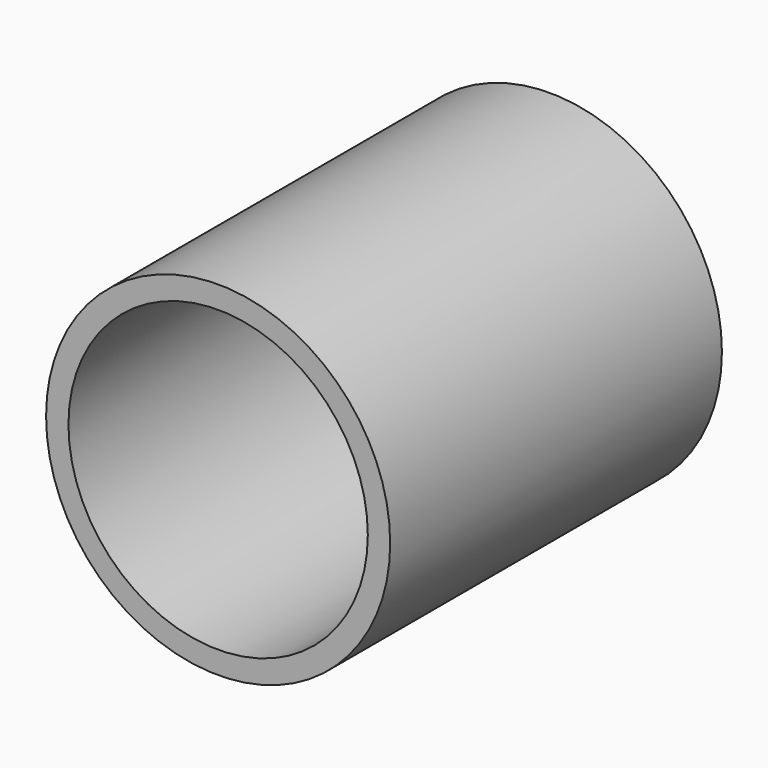
from build123d import *

# Parameters (mm, degrees)
F0_R     = 42.1551609163
F0_R_2   = 36.6737913898
F1_DEPTH = 101.6
F2_R     = 36.6906853339
F3_DEPTH = 0.254


# Not quite as in the source:
# - the program builds the solid bodies; features that only make, move or delete a surface that nothing else refers to are left out


with BuildPart() as f1:
    # F0 (on Front) → F1 (new body)
    with BuildSketch(Plane.XZ):
        Circle(F0_R)
        Circle(F0_R_2, mode=Mode.SUBTRACT)
    extrude(amount=-F1_DEPTH)

    # F2 (on face) → F3 (join)
    with BuildSketch(Plane(origin=(0, 101.6, 0), x_dir=(-1, 0, 0), z_dir=(0, 1, 0))):
        Circle(F2_R)
    extrude(amount=F3_DEPTH)


solid = f1.part
